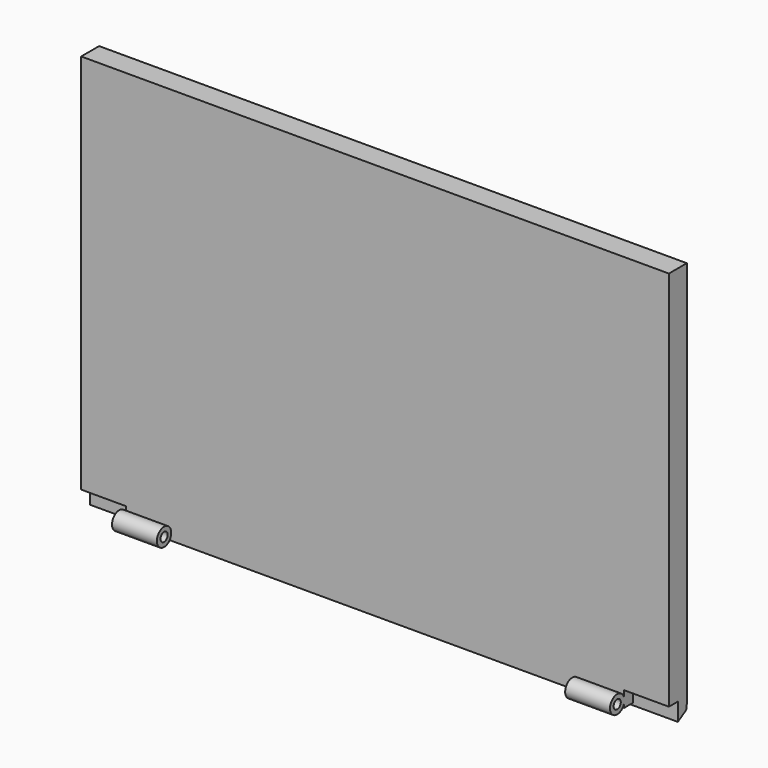
from build123d import *

# Parameters (mm, degrees)
F0_W        = 131
F0_H        = 89
F1_DEPTH    = 5
F3_START    = -10
F2_R        = 2
F2_R_2      = 1
F3_DEPTH    = 10
F5_START    = -10
F4_R        = 2
F4_R_2      = 1
F5_DEPTH    = 10
F6_W        = 111
F6_H        = 0.5
F7_DEPTH    = 2.5
F8_T1_DEPTH = 152.6506350946


# Not quite as in the source:
# - a fillet or chamfer that OpenCascade refuses, or shapes differently, is made with other operations: its cross-section is extruded or revolved along the edge and cut away or added


with BuildPart() as f1:
    # F0 (on Front) → F1 (new body)
    with BuildSketch(Plane.XZ):
        Rectangle(F0_W, F0_H)
    extrude(amount=F1_DEPTH)

    # F2 (on face) → F3 (join)
    with BuildSketch(Plane(origin=(-65.5, 0, 0), x_dir=(0, -1, 0), z_dir=(-1, 0, 0)).offset(F3_START)):
        with Locations((6.9, -42.5)):
            Circle(F2_R)
        with Locations((6.9, -42.5)):
            Circle(F2_R_2, mode=Mode.SUBTRACT)
    extrude(amount=-F3_DEPTH)

    # F4 (on face) → F5 (join)
    with BuildSketch(Plane.YZ.offset(65.5).offset(F5_START)):
        with Locations((-6.9, -42.5)):
            Circle(F4_R)
        with Locations((-6.9, -42.5)):
            Circle(F4_R_2, mode=Mode.SUBTRACT)
    extrude(amount=-F5_DEPTH)

    # F6 (on face) → F7 (cut)
    with BuildSketch(Plane.XZ.offset(5)):
        Polygon((55.5, -44.5), (65.5, -44.5), (65.5, -40.5), (55.5, -40.5), (55.5, -44), align=None)
        with Locations((0, -44.25)):
            Rectangle(F6_W, F6_H)
        Polygon((-65.5, -44.5), (-55.5, -44.5), (-55.5, -44), (-55.5, -40.5), (-65.5, -40.5), align=None)
    extrude(amount=-F7_DEPTH, mode=Mode.SUBTRACT)

    # F8: fillet of radius 5 on 1 edges, made by hand

    # F8_s2 → F8_t1 (cut)
    with BuildSketch(Plane.YZ.offset(-76.3253175473)):
        with BuildLine():
            add(Edge.make_bspline(
                [(0, -40.1698729811), (0, -43.056624327), (-2.5, -44.5)],
                knots=[0, 0, 0, 1, 1, 1], degree=2, weights=[1, 9, 1]))
            Line((-2.5, -44.5), (0, -44.5))
            Line((0, -44.5), (0, -40.1698729811))
        make_face()
    extrude(amount=F8_T1_DEPTH, mode=Mode.SUBTRACT)


solid = f1.part
